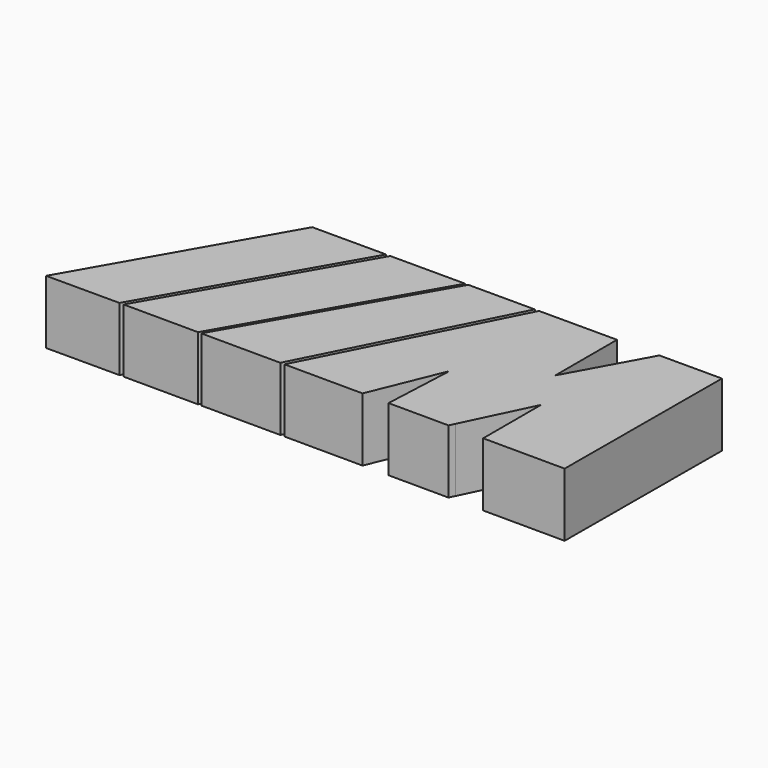
from build123d import *

# Parameters (mm, degrees)
F1_DEPTH = 4.5


# Not quite as in the source:
# - a feature names something its author has since deleted; it is built from what else it names


with BuildPart() as f1:
    # F0 (on Top) → F1 (new body)
    with BuildSketch(Plane.XY):
        Polygon((-3.4254482334, 6.7703626119), (-7.8505282334, 6.7703626119), (-10.8505282334, 1.3056819865), (-10.8505282334, 6.7703626119), (-16.3737182334, 6.7703626119), (-23.3664704371, -7.0105993377), (-17.822726575, -7.0309609225), (-15.7404388942, -1.9405601371), (-15.978364491, -7.0377350693), (-11.7246839348, -7.053358388), (-11.5361148701, -6.6621245411), (-9.2622392988, -1.9443990291), (-9.2622392988, -7.0624026867), (-3.4763325698, -7.08365371), align=None)
    extrude(amount=F1_DEPTH)


with BuildPart() as f1b:
    # F0 (on Top) → F1, piece 2 (new body)
    with BuildSketch(Plane.XY):
        Polygon((-32.4264727533, 6.7703626119), (-40.2658395469, -6.9485297427), (-40.2772985399, -6.9675564117), (-35.0855463293, -6.9675564117), (-27.203282851, 6.7703626119), align=None)
    extrude(amount=F1_DEPTH)


with BuildPart() as f1c:
    # F0 (on Top) → F1, piece 3 (new body)
    with BuildSketch(Plane.XY):
        Polygon((-21.6101612896, 6.7703626119), (-26.903282851, 6.7703626119), (-34.7861772074, -6.9686559628), (-29.5041866934, -6.9880561552), align=None)
    extrude(amount=F1_DEPTH)


with BuildPart() as f1d:
    # F0 (on Top) → F1, piece 4 (new body)
    with BuildSketch(Plane.XY):
        Polygon((-16.6737182334, 6.7703626119), (-21.380092851, 6.7703626119), (-29.2746020719, -6.9888993952), (-23.6659123659, -7.0094995192), align=None)
    extrude(amount=F1_DEPTH)


solid = Compound([f1.part, f1b.part, f1c.part, f1d.part])
